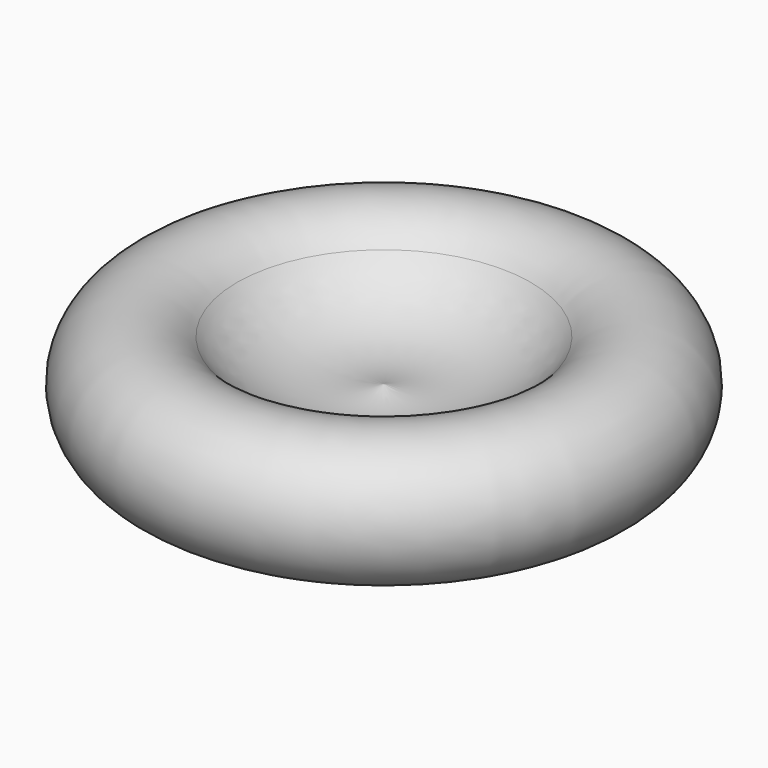
from build123d import *


# Not quite as in the source:
# - a feature of the source that left no trace in its solid (it failed there, or was rolled back) is left out


with BuildPart() as f1:
    # F0 (on Front) → F1 (revolve)
    with BuildSketch(Plane.XZ):
        with BuildLine():
            ThreePointArc((0, 5), (-6.0592152712, 4.825669304), (-11.1231341484, 8.1575166142))
            ThreePointArc((-11.1231341484, 8.1575166142), (-19.5159485754, 7.1462079267), (-15, 0))
            Line((-15, 0), (0, 0))
            Line((0, 0), (0, 5))
        make_face()
    revolve(axis=Axis((0, 0, 2.5), (0, 0, 1)))


solid = f1.part
